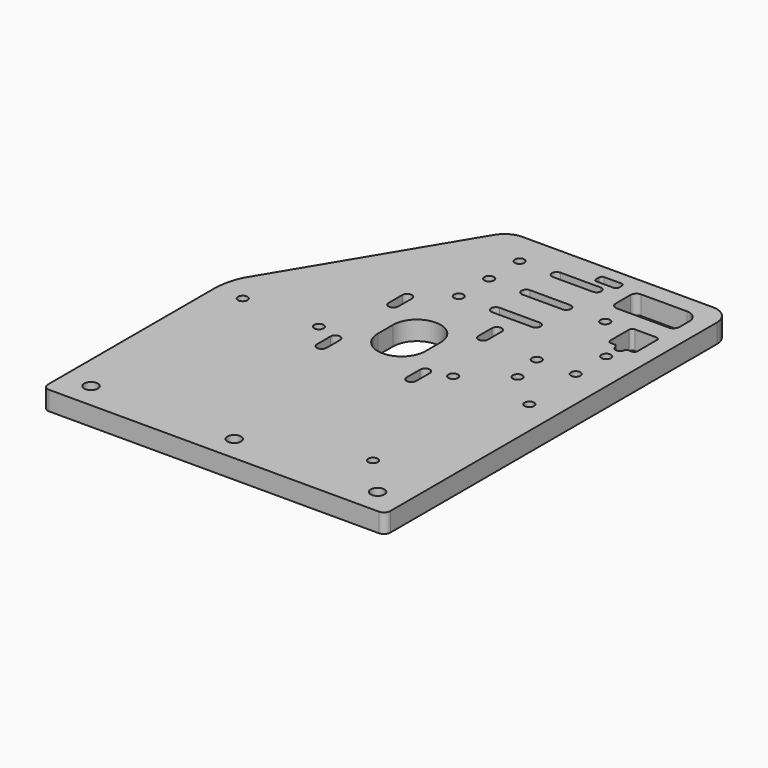
from build123d import *

# Parameters (mm, degrees)
F0_R     = 4.6
F0_R_2   = 2.5
F0_R_3   = 3.6
F1_DEPTH = 10
F2_DEPTH = 4


# Not quite as in the source:
# - ends of sketch curves that miss each other by under 0.0002 mm in the source are joined


with BuildPart() as f1:
    # F0 (on Top) → F1 (new body)
    with BuildSketch(Plane.XY):
        with BuildLine():
            ThreePointArc((-90.000003, -110.40631), (-89.0264648164, -112.7715584011), (-86.6700030006, -113.7661760688))
            Line((-86.6700030006, -113.7661760688), (86.639997, -113.766176))
            ThreePointArc((86.639997, -113.766176), (89.0158757848, -112.7820547848), (89.999997, -110.406176))
            Line((89.999997, -110.406176), (89.999997, 104.053824))
            ThreePointArc((89.999997, 104.053824), (87.1712591943, 110.8980101257), (80.330002, 113.733824))
            Line((80.330002, 113.733824), (-18.849998, 113.733824))
            ThreePointArc((-18.849998, 113.733824), (-25.2573363418, 112.4191498026), (-30.0255163302, 107.9417831984))
            Line((-30.0255163302, 107.9417831984), (-86.679704, 13.65338))
            ThreePointArc((-86.679704, 13.65338), (-89.1601424865, 6.2787905251), (-90.000003, -1.45631))
            Line((-90.000003, -1.45631), (-90.000003, -110.40631))
        make_face()
        with Locations((-75.300003, -100.436176)):
            Circle(F0_R, mode=Mode.SUBTRACT)
        with Locations((-3e-06, -100.436176)):
            Circle(F0_R, mode=Mode.SUBTRACT)
        with Locations((-75.300003, -0.736176)):
            Circle(F0_R, mode=Mode.SUBTRACT)
        with Locations((-35.300003, -0.736176)):
            Circle(F0_R, mode=Mode.SUBTRACT)
        with BuildLine():
            ThreePointArc((-18.930003, -13.556176), (-23.570003, -18.196176), (-28.210003, -13.556176))
            Line((-28.210003, -13.556176), (-28.210003, -4.556176))
            ThreePointArc((-28.210003, -4.556176), (-23.570003, 0.083824), (-18.930003, -4.556176))
            Line((-18.930003, -4.556176), (-18.930003, -13.556176))
        make_face(mode=Mode.SUBTRACT)
        with Locations((75.299997, -100.436176)):
            Circle(F0_R, mode=Mode.SUBTRACT)
        with Locations((56.339997, -79.736176)):
            Circle(F0_R_2, mode=Mode.SUBTRACT)
        with BuildLine():
            ThreePointArc((18.929997, -4.556176), (23.569997, 0.083824), (28.209997, -4.556176))
            Line((28.209997, -4.556176), (28.209997, -13.556176))
            ThreePointArc((28.209997, -13.556176), (23.569997, -18.196176), (18.929997, -13.556176))
            Line((18.929997, -13.556176), (18.929997, -4.556176))
        make_face(mode=Mode.SUBTRACT)
        with Locations((35.299997, -0.736176)):
            Circle(F0_R, mode=Mode.SUBTRACT)
        with Locations((75.299997, -0.736176)):
            Circle(F0_R, mode=Mode.SUBTRACT)
        with BuildLine():
            ThreePointArc((12.499997, 9.513824), (-3e-06, -2.986176), (-12.500003, 9.513824))
            Line((-12.500003, 9.513824), (-12.500003, 19.513824))
            ThreePointArc((-12.500003, 19.513824), (-3e-06, 32.013824), (12.499997, 19.513824))
            Line((12.499997, 19.513824), (12.499997, 9.513824))
        make_face(mode=Mode.SUBTRACT)
        with BuildLine():
            ThreePointArc((-28.210003, 42.583824), (-23.570003, 47.223824), (-18.930003, 42.583824))
            Line((-18.930003, 42.583824), (-18.930003, 33.583824))
            ThreePointArc((-18.930003, 33.583824), (-23.570003, 28.943824), (-28.210003, 33.583824))
            Line((-28.210003, 33.583824), (-28.210003, 42.583824))
        make_face(mode=Mode.SUBTRACT)
        with Locations((-7.310003, 56.173824)):
            Circle(F0_R_2, mode=Mode.SUBTRACT)
        with Locations((-7.310003, 76.173824)):
            Circle(F0_R_2, mode=Mode.SUBTRACT)
        with Locations((-7.310003, 96.173824)):
            Circle(F0_R_2, mode=Mode.SUBTRACT)
        with BuildLine():
            ThreePointArc((28.209997, 33.583824), (23.569997, 28.943824), (18.929997, 33.583824))
            Line((18.929997, 33.583824), (18.929997, 42.583824))
            ThreePointArc((18.929997, 42.583824), (23.569997, 47.223824), (28.209997, 42.583824))
            Line((28.209997, 42.583824), (28.209997, 33.583824))
        make_face(mode=Mode.SUBTRACT)
        with BuildLine():
            ThreePointArc((12.189997, 51.573824), (7.589997, 56.173824), (12.189997, 60.773824))
            Line((12.189997, 60.773824), (33.189997, 60.773824))
            ThreePointArc((33.189997, 60.773824), (37.789997, 56.173824), (33.189997, 51.573824))
            Line((33.189997, 51.573824), (12.189997, 51.573824))
        make_face(mode=Mode.SUBTRACT)
        with Locations((56.339997, 15.263824)):
            Circle(F0_R_2, mode=Mode.SUBTRACT)
        with Locations((52.849997, 32.213824)):
            Circle(F0_R_2, mode=Mode.SUBTRACT)
        with Locations((73.349997, 32.213824)):
            Circle(F0_R, mode=Mode.SUBTRACT)
        with Locations((73.349997, 52.213824)):
            Circle(F0_R, mode=Mode.SUBTRACT)
        with BuildLine():
            ThreePointArc((12.189997, 71.573824), (7.589997, 76.173824), (12.189997, 80.773824))
            Line((12.189997, 80.773824), (33.189997, 80.773824))
            ThreePointArc((33.189997, 80.773824), (37.789997, 76.173824), (33.189997, 71.573824))
            Line((33.189997, 71.573824), (12.189997, 71.573824))
        make_face(mode=Mode.SUBTRACT)
        with BuildLine():
            ThreePointArc((12.189997, 91.573824), (7.589997, 96.173824), (12.189997, 100.773824))
            Line((12.189997, 100.773824), (33.189997, 100.773824))
            ThreePointArc((33.189997, 100.773824), (37.789997, 96.173824), (33.189997, 91.573824))
            Line((33.189997, 91.573824), (12.189997, 91.573824))
        make_face(mode=Mode.SUBTRACT)
        with BuildLine():
            ThreePointArc((28.629997, 101.763824), (27.6117632351, 102.1855902351), (27.189997, 103.203824))
            Line((27.189997, 103.203824), (27.189997, 105.323824))
            ThreePointArc((27.189997, 105.323824), (27.6117632351, 106.3420577649), (28.629997, 106.763824))
            Line((28.629997, 106.763824), (37.749997, 106.763824))
            ThreePointArc((37.749997, 106.763824), (38.7682307649, 106.3420577649), (39.189997, 105.323824))
            Line((39.189997, 105.323824), (39.189997, 103.203824))
            ThreePointArc((39.189997, 103.203824), (38.7682307649, 102.1855902351), (37.749997, 101.763824))
            Line((37.749997, 101.763824), (28.629997, 101.763824))
        make_face(mode=Mode.SUBTRACT)
        with Locations((53.689997, 76.173824)):
            Circle(F0_R_2, mode=Mode.SUBTRACT)
        with BuildLine():
            Line((78.839997, 62.193824), (76.369997, 62.193824))
            Line((76.369997, 62.193824), (75.802984, 61.483539))
            add(Edge.make_bspline(
                [(70.89701, 61.4835398497), (70.8970091503, 59.0305524249), (73.3499965751, 59.030552), (75.802984, 59.0305515751), (75.802984, 61.483539)],
                knots=[3.1415923072, 3.1415923072, 3.1415923072, 4.7123888072, 4.7123888072, 6.2831853072, 6.2831853072, 6.2831853072], degree=2, weights=[1, 0.7071067199, 1, 0.7071067199, 1]))
            Line((70.89701, 61.4835398497), (69.929997, 62.694895))
            Line((69.929997, 62.694895), (67.459997, 62.694895))
            ThreePointArc((67.459997, 62.694895), (66.2861997432, 63.1810977432), (65.799997, 64.354895))
            Line((65.799997, 64.354895), (65.799997, 76.683824))
            ThreePointArc((65.799997, 76.683824), (66.2861997432, 77.8576212568), (67.459997, 78.343824))
            Line((67.459997, 78.343824), (78.839997, 78.343824))
            ThreePointArc((78.839997, 78.343824), (80.0137942568, 77.8576212568), (80.499997, 76.683824))
            Line((80.499997, 76.683824), (80.499997, 63.853824))
            ThreePointArc((80.499997, 63.853824), (80.0137942568, 62.6800267432), (78.839997, 62.193824))
        make_face(mode=Mode.SUBTRACT)
        with BuildLine():
            ThreePointArc((50.139997, 88.263824), (47.9196817071, 89.1835087071), (46.999997, 91.403824))
            Line((46.999997, 91.403824), (46.999997, 101.093824))
            ThreePointArc((46.999997, 101.093824), (47.9196817071, 103.3141392929), (50.139997, 104.233824))
            Line((50.139997, 104.233824), (74.149997, 104.233824))
            ThreePointArc((74.149997, 104.233824), (78.6401250605, 102.3739520605), (80.499997, 97.883824))
            Line((80.499997, 97.883824), (80.499997, 91.403824))
            ThreePointArc((80.499997, 91.403824), (79.5803122929, 89.1835087071), (77.359997, 88.263824))
            Line((77.359997, 88.263824), (50.139997, 88.263824))
        make_face(mode=Mode.SUBTRACT)
        with Locations((-75.300003, -0.736176)):
            Circle(F0_R)
        with Locations((-75.300003, -0.736176)):
            Circle(F0_R_2, mode=Mode.SUBTRACT)
        with Locations((-35.300003, -0.736176)):
            Circle(F0_R)
        with Locations((-35.300003, -0.736176)):
            Circle(F0_R_2, mode=Mode.SUBTRACT)
        with BuildLine():
            Line((-28.210003, -4.556176), (-28.210003, -13.556176))
            ThreePointArc((-28.210003, -13.556176), (-23.570003, -18.196176), (-18.930003, -13.556176))
            Line((-18.930003, -13.556176), (-18.930003, -4.556176))
            ThreePointArc((-18.930003, -4.556176), (-23.570003, 0.083824), (-28.210003, -4.556176))
        make_face()
        with BuildLine():
            ThreePointArc((-21.030003, -13.556176), (-23.570003, -16.096176), (-26.110003, -13.556176))
            Line((-26.110003, -13.556176), (-26.110003, -4.556176))
            ThreePointArc((-26.110003, -4.556176), (-23.570003, -2.016176), (-21.030003, -4.556176))
            Line((-21.030003, -4.556176), (-21.030003, -13.556176))
        make_face(mode=Mode.SUBTRACT)
        with BuildLine():
            Line((-18.930003, 33.583824), (-18.930003, 42.583824))
            ThreePointArc((-18.930003, 42.583824), (-23.570003, 47.223824), (-28.210003, 42.583824))
            Line((-28.210003, 42.583824), (-28.210003, 33.583824))
            ThreePointArc((-28.210003, 33.583824), (-23.570003, 28.943824), (-18.930003, 33.583824))
        make_face()
        with BuildLine():
            ThreePointArc((-21.030003, 33.583824), (-23.570003, 31.043824), (-26.110003, 33.583824))
            Line((-26.110003, 33.583824), (-26.110003, 42.583824))
            ThreePointArc((-26.110003, 42.583824), (-23.570003, 45.123824), (-21.030003, 42.583824))
            Line((-21.030003, 42.583824), (-21.030003, 33.583824))
        make_face(mode=Mode.SUBTRACT)
        with BuildLine():
            Line((18.929997, 42.583824), (18.929997, 33.583824))
            ThreePointArc((18.929997, 33.583824), (23.569997, 28.943824), (28.209997, 33.583824))
            Line((28.209997, 33.583824), (28.209997, 42.583824))
            ThreePointArc((28.209997, 42.583824), (23.569997, 47.223824), (18.929997, 42.583824))
        make_face()
        with BuildLine():
            ThreePointArc((26.109997, 33.583824), (23.569997, 31.043824), (21.029997, 33.583824))
            Line((21.029997, 33.583824), (21.029997, 42.583824))
            ThreePointArc((21.029997, 42.583824), (23.569997, 45.123824), (26.109997, 42.583824))
            Line((26.109997, 42.583824), (26.109997, 33.583824))
        make_face(mode=Mode.SUBTRACT)
        with BuildLine():
            Line((28.209997, -13.556176), (28.209997, -4.556176))
            ThreePointArc((28.209997, -4.556176), (23.569997, 0.083824), (18.929997, -4.556176))
            Line((18.929997, -4.556176), (18.929997, -13.556176))
            ThreePointArc((18.929997, -13.556176), (23.569997, -18.196176), (28.209997, -13.556176))
        make_face()
        with BuildLine():
            ThreePointArc((26.109997, -13.556176), (23.569997, -16.096176), (21.029997, -13.556176))
            Line((21.029997, -13.556176), (21.029997, -4.556176))
            ThreePointArc((21.029997, -4.556176), (23.569997, -2.016176), (26.109997, -4.556176))
            Line((26.109997, -4.556176), (26.109997, -13.556176))
        make_face(mode=Mode.SUBTRACT)
        with Locations((35.299997, -0.736176)):
            Circle(F0_R)
        with Locations((35.299997, -0.736176)):
            Circle(F0_R_2, mode=Mode.SUBTRACT)
        with Locations((75.299997, -0.736176)):
            Circle(F0_R)
        with Locations((75.299997, -0.736176)):
            Circle(F0_R_2, mode=Mode.SUBTRACT)
        with Locations((-75.300003, -100.436176)):
            Circle(F0_R)
        with Locations((-75.300003, -100.436176)):
            Circle(F0_R_3, mode=Mode.SUBTRACT)
        with Locations((-3e-06, -100.436176)):
            Circle(F0_R)
        with Locations((-3e-06, -100.436176)):
            Circle(F0_R_3, mode=Mode.SUBTRACT)
        with Locations((75.299997, -100.436176)):
            Circle(F0_R)
        with Locations((75.299997, -100.436176)):
            Circle(F0_R_3, mode=Mode.SUBTRACT)
        with BuildLine():
            Line((33.189997, 60.773824), (12.189997, 60.773824))
            ThreePointArc((12.189997, 60.773824), (7.589997, 56.173824), (12.189997, 51.573824))
            Line((12.189997, 51.573824), (33.189997, 51.573824))
            ThreePointArc((33.189997, 51.573824), (37.789997, 56.173824), (33.189997, 60.773824))
        make_face()
        with BuildLine():
            ThreePointArc((33.189997, 58.673824), (35.689997, 56.173824), (33.189997, 53.673824))
            Line((33.189997, 53.673824), (12.189997, 53.673824))
            ThreePointArc((12.189997, 53.673824), (9.689997, 56.173824), (12.189997, 58.673824))
            Line((12.189997, 58.673824), (33.189997, 58.673824))
        make_face(mode=Mode.SUBTRACT)
        with BuildLine():
            Line((33.189997, 80.773824), (12.189997, 80.773824))
            ThreePointArc((12.189997, 80.773824), (7.589997, 76.173824), (12.189997, 71.573824))
            Line((12.189997, 71.573824), (33.189997, 71.573824))
            ThreePointArc((33.189997, 71.573824), (37.789997, 76.173824), (33.189997, 80.773824))
        make_face()
        with BuildLine():
            ThreePointArc((33.189997, 78.673824), (35.689997, 76.173824), (33.189997, 73.673824))
            Line((33.189997, 73.673824), (12.189997, 73.673824))
            ThreePointArc((12.189997, 73.673824), (9.689997, 76.173824), (12.189997, 78.673824))
            Line((12.189997, 78.673824), (33.189997, 78.673824))
        make_face(mode=Mode.SUBTRACT)
        with BuildLine():
            Line((33.189997, 100.773824), (12.189997, 100.773824))
            ThreePointArc((12.189997, 100.773824), (7.589997, 96.173824), (12.189997, 91.573824))
            Line((12.189997, 91.573824), (33.189997, 91.573824))
            ThreePointArc((33.189997, 91.573824), (37.789997, 96.173824), (33.189997, 100.773824))
        make_face()
        with BuildLine():
            ThreePointArc((33.189997, 98.673824), (35.689997, 96.173824), (33.189997, 93.673824))
            Line((33.189997, 93.673824), (12.189997, 93.673824))
            ThreePointArc((12.189997, 93.673824), (9.689997, 96.173824), (12.189997, 98.673824))
            Line((12.189997, 98.673824), (33.189997, 98.673824))
        make_face(mode=Mode.SUBTRACT)
        with Locations((73.349997, 32.213824)):
            Circle(F0_R)
        with Locations((73.349997, 32.213824)):
            Circle(F0_R_2, mode=Mode.SUBTRACT)
        with Locations((73.349997, 52.213824)):
            Circle(F0_R)
        with Locations((73.349997, 52.213824)):
            Circle(F0_R_2, mode=Mode.SUBTRACT)
    extrude(amount=F1_DEPTH)

    # F0 (on Top) → F2 (cut, through all)
    with BuildSketch(Plane.XY):
        with Locations((-75.300003, -100.436176)):
            Circle(F0_R)
        with Locations((-75.300003, -100.436176)):
            Circle(F0_R_3, mode=Mode.SUBTRACT)
        with Locations((-3e-06, -100.436176)):
            Circle(F0_R)
        with Locations((-3e-06, -100.436176)):
            Circle(F0_R_3, mode=Mode.SUBTRACT)
        with Locations((75.299997, -100.436176)):
            Circle(F0_R)
        with Locations((75.299997, -100.436176)):
            Circle(F0_R_3, mode=Mode.SUBTRACT)
        with BuildLine():
            Line((-28.210003, -4.556176), (-28.210003, -13.556176))
            ThreePointArc((-28.210003, -13.556176), (-23.570003, -18.196176), (-18.930003, -13.556176))
            Line((-18.930003, -13.556176), (-18.930003, -4.556176))
            ThreePointArc((-18.930003, -4.556176), (-23.570003, 0.083824), (-28.210003, -4.556176))
        make_face()
        with BuildLine():
            ThreePointArc((-21.030003, -13.556176), (-23.570003, -16.096176), (-26.110003, -13.556176))
            Line((-26.110003, -13.556176), (-26.110003, -4.556176))
            ThreePointArc((-26.110003, -4.556176), (-23.570003, -2.016176), (-21.030003, -4.556176))
            Line((-21.030003, -4.556176), (-21.030003, -13.556176))
        make_face(mode=Mode.SUBTRACT)
        with BuildLine():
            Line((28.209997, -13.556176), (28.209997, -4.556176))
            ThreePointArc((28.209997, -4.556176), (23.569997, 0.083824), (18.929997, -4.556176))
            Line((18.929997, -4.556176), (18.929997, -13.556176))
            ThreePointArc((18.929997, -13.556176), (23.569997, -18.196176), (28.209997, -13.556176))
        make_face()
        with BuildLine():
            ThreePointArc((26.109997, -13.556176), (23.569997, -16.096176), (21.029997, -13.556176))
            Line((21.029997, -13.556176), (21.029997, -4.556176))
            ThreePointArc((21.029997, -4.556176), (23.569997, -2.016176), (26.109997, -4.556176))
            Line((26.109997, -4.556176), (26.109997, -13.556176))
        make_face(mode=Mode.SUBTRACT)
        with BuildLine():
            Line((-18.930003, 33.583824), (-18.930003, 42.583824))
            ThreePointArc((-18.930003, 42.583824), (-23.570003, 47.223824), (-28.210003, 42.583824))
            Line((-28.210003, 42.583824), (-28.210003, 33.583824))
            ThreePointArc((-28.210003, 33.583824), (-23.570003, 28.943824), (-18.930003, 33.583824))
        make_face()
        with BuildLine():
            ThreePointArc((-21.030003, 33.583824), (-23.570003, 31.043824), (-26.110003, 33.583824))
            Line((-26.110003, 33.583824), (-26.110003, 42.583824))
            ThreePointArc((-26.110003, 42.583824), (-23.570003, 45.123824), (-21.030003, 42.583824))
            Line((-21.030003, 42.583824), (-21.030003, 33.583824))
        make_face(mode=Mode.SUBTRACT)
        with BuildLine():
            Line((18.929997, 42.583824), (18.929997, 33.583824))
            ThreePointArc((18.929997, 33.583824), (23.569997, 28.943824), (28.209997, 33.583824))
            Line((28.209997, 33.583824), (28.209997, 42.583824))
            ThreePointArc((28.209997, 42.583824), (23.569997, 47.223824), (18.929997, 42.583824))
        make_face()
        with BuildLine():
            ThreePointArc((26.109997, 33.583824), (23.569997, 31.043824), (21.029997, 33.583824))
            Line((21.029997, 33.583824), (21.029997, 42.583824))
            ThreePointArc((21.029997, 42.583824), (23.569997, 45.123824), (26.109997, 42.583824))
            Line((26.109997, 42.583824), (26.109997, 33.583824))
        make_face(mode=Mode.SUBTRACT)
        with Locations((-75.300003, -0.736176)):
            Circle(F0_R)
        with Locations((-75.300003, -0.736176)):
            Circle(F0_R_2, mode=Mode.SUBTRACT)
        with Locations((35.299997, -0.736176)):
            Circle(F0_R)
        with Locations((35.299997, -0.736176)):
            Circle(F0_R_2, mode=Mode.SUBTRACT)
        with Locations((-35.300003, -0.736176)):
            Circle(F0_R)
        with Locations((-35.300003, -0.736176)):
            Circle(F0_R_2, mode=Mode.SUBTRACT)
        with Locations((75.299997, -0.736176)):
            Circle(F0_R)
        with Locations((75.299997, -0.736176)):
            Circle(F0_R_2, mode=Mode.SUBTRACT)
        with Locations((73.349997, 32.213824)):
            Circle(F0_R)
        with Locations((73.349997, 32.213824)):
            Circle(F0_R_2, mode=Mode.SUBTRACT)
        with Locations((73.349997, 52.213824)):
            Circle(F0_R)
        with Locations((73.349997, 52.213824)):
            Circle(F0_R_2, mode=Mode.SUBTRACT)
        with BuildLine():
            Line((33.189997, 60.773824), (12.189997, 60.773824))
            ThreePointArc((12.189997, 60.773824), (7.589997, 56.173824), (12.189997, 51.573824))
            Line((12.189997, 51.573824), (33.189997, 51.573824))
            ThreePointArc((33.189997, 51.573824), (37.789997, 56.173824), (33.189997, 60.773824))
        make_face()
        with BuildLine():
            ThreePointArc((33.189997, 58.673824), (35.689997, 56.173824), (33.189997, 53.673824))
            Line((33.189997, 53.673824), (12.189997, 53.673824))
            ThreePointArc((12.189997, 53.673824), (9.689997, 56.173824), (12.189997, 58.673824))
            Line((12.189997, 58.673824), (33.189997, 58.673824))
        make_face(mode=Mode.SUBTRACT)
        with BuildLine():
            Line((33.189997, 80.773824), (12.189997, 80.773824))
            ThreePointArc((12.189997, 80.773824), (7.589997, 76.173824), (12.189997, 71.573824))
            Line((12.189997, 71.573824), (33.189997, 71.573824))
            ThreePointArc((33.189997, 71.573824), (37.789997, 76.173824), (33.189997, 80.773824))
        make_face()
        with BuildLine():
            ThreePointArc((33.189997, 78.673824), (35.689997, 76.173824), (33.189997, 73.673824))
            Line((33.189997, 73.673824), (12.189997, 73.673824))
            ThreePointArc((12.189997, 73.673824), (9.689997, 76.173824), (12.189997, 78.673824))
            Line((12.189997, 78.673824), (33.189997, 78.673824))
        make_face(mode=Mode.SUBTRACT)
        with BuildLine():
            Line((33.189997, 100.773824), (12.189997, 100.773824))
            ThreePointArc((12.189997, 100.773824), (7.589997, 96.173824), (12.189997, 91.573824))
            Line((12.189997, 91.573824), (33.189997, 91.573824))
            ThreePointArc((33.189997, 91.573824), (37.789997, 96.173824), (33.189997, 100.773824))
        make_face()
        with BuildLine():
            ThreePointArc((33.189997, 98.673824), (35.689997, 96.173824), (33.189997, 93.673824))
            Line((33.189997, 93.673824), (12.189997, 93.673824))
            ThreePointArc((12.189997, 93.673824), (9.689997, 96.173824), (12.189997, 98.673824))
            Line((12.189997, 98.673824), (33.189997, 98.673824))
        make_face(mode=Mode.SUBTRACT)
    extrude(amount=F2_DEPTH, mode=Mode.SUBTRACT)


solid = f1.part
